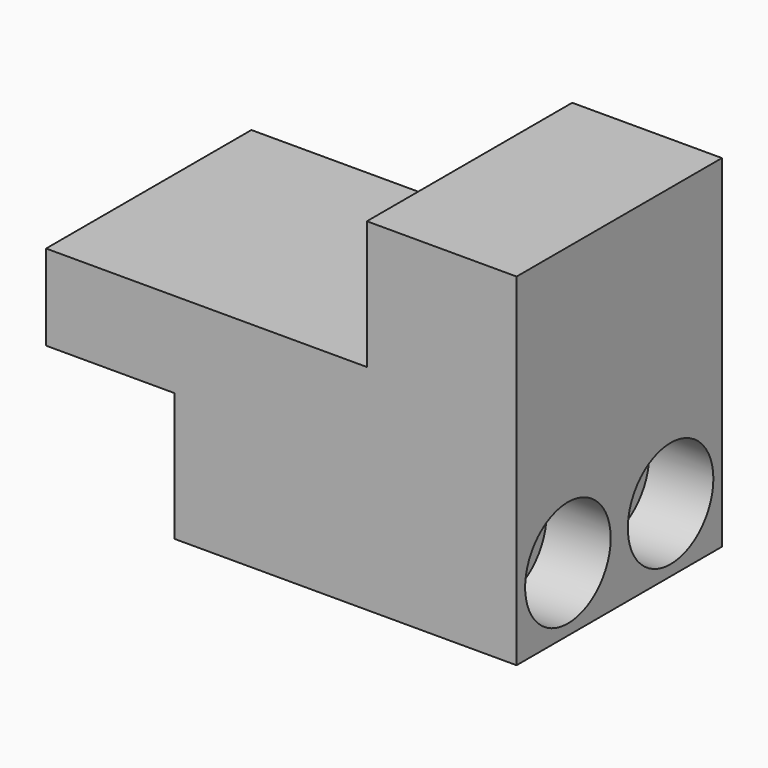
from build123d import *

# Parameters (mm, degrees)
F1_DEPTH       = 19.05
F3_D           = 9.525
F3_CBORE_D     = 15.875
F3_CBORE_DEPTH = 9.525


# Not quite as in the source:
# - a length typed as a fraction of an inch, garbled in the dataset ("3 / 203.2 mm" for 3/8 in), is restored


with BuildPart() as f1:
    # F0 (on Front) → F1 (new body, symmetric)
    with BuildSketch(Plane.XZ):
        Polygon((-50.8, 0), (0, 0), (0, 50.8), (-22.225, 50.8), (-22.225, 31.75), (-69.85, 31.75), (-69.85, 19.05), (-50.8, 19.05), align=None)
    extrude(amount=F1_DEPTH, both=True)

    # F3 (through all)
    with Locations(Plane.YZ):
        with Locations((-9.525, 9.525), (9.525, 9.525)):
            CounterBoreHole(F3_D / 2, F3_CBORE_D / 2, F3_CBORE_DEPTH)


solid = f1.part
